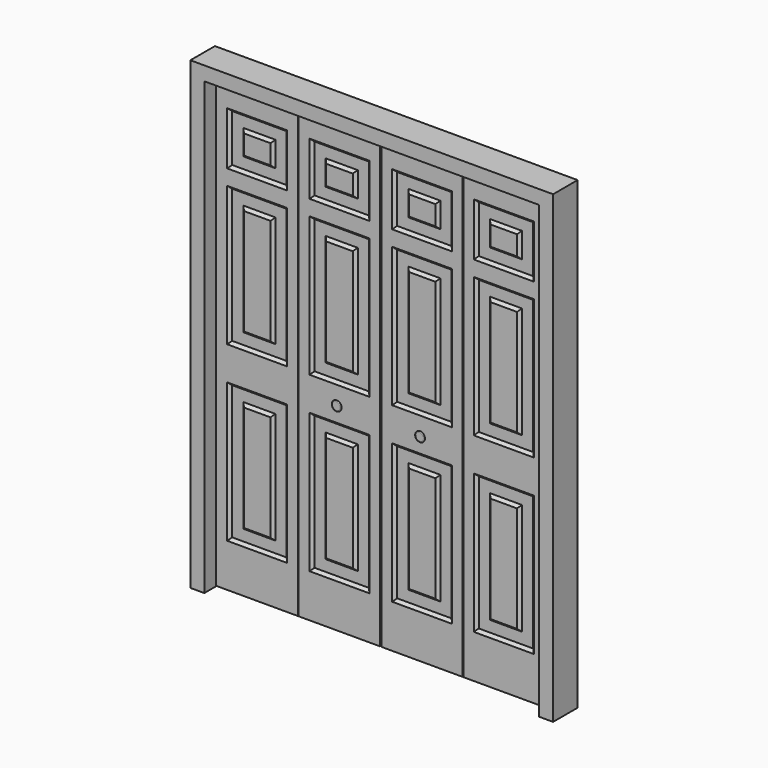
from build123d import *

# Parameters (mm, degrees)
F1_DEPTH  = 69.85
F0_W      = 1524
F0_H      = 2051.05
F2_DEPTH  = 19.05
F3_W      = 520.9721539497
F3_H      = 12.7
F4_DEPTH  = 88.901
F5_W      = 3.175
F5_H      = 2025.65
F7_DEPTH  = 88.901
F5_W_2    = 247.65
F5_H_2    = 215.9
F5_W_3    = 146.05
F5_H_3    = 114.3
F5_H_4    = 609.6
F5_H_5    = 508
F6_W      = 247.65
F6_H      = 215.9
F6_W_2    = 146.05
F6_H_2    = 114.3
F6_H_3    = 609.6
F6_H_4    = 508
F8_DEPTH  = 12.7
F9_SIZE   = 12.69999
F10_SIZE  = 12.69999
F11_R     = 6.35
F12_DEPTH = 12.7
F13_R     = 22.225
F14_DEPTH = 3.175
F15_R     = 6.35
F16_DEPTH = 12.7
F17_R     = 22.225
F18_DEPTH = 3.175


# Not quite as in the source:
# - a fillet or chamfer that OpenCascade refuses, or shapes differently, is made with other operations: its cross-section is extruded or revolved along the edge and cut away or added
# - a fillet or chamfer is up to 0.001 mm smaller than in the source, because OpenCascade refuses the exact size


with BuildPart() as f1:
    # F0 (on Front) → F1 (new body, symmetric)
    with BuildSketch(Plane.XZ):
        Polygon((825.5, 1057.275), (-825.5, 1057.275), (-825.5, -1057.275), (-762, -1057.275), (-762, 993.775), (762, 993.775), (762, -1057.275), (825.5, -1057.275), align=None)
    extrude(amount=F1_DEPTH, both=True)

    # F0 (on Front) → F2 (join, symmetric)
    with BuildSketch(Plane.XZ):
        with Locations((0, -31.75)):
            Rectangle(F0_W, F0_H)
    extrude(amount=F2_DEPTH, both=True)

    # F3 (on face) → F4 (cut, through all)
    with BuildSketch(Plane.XZ.offset(19.05)):
        Polygon((0, 981.075), (-3.175, 981.075), (-3.175, -1044.575), (0, -1044.575), (3.175, -1044.575), (3.175, 981.075), align=None)
        Polygon((-3.175, -1044.575), (-749.3, -1044.575), (-749.3, 981.075), (-683.8496296883, 981.075), (-683.8496296883, 993.775), (-762, 993.775), (-762, -1057.275), (762, -1057.275), (762, 993.775), (683.8496296883, 993.775), (683.8496296883, 981.075), (749.3, 981.075), (749.3, -1044.575), (3.175, -1044.575), (0, -1044.575), align=None)
        with Locations((410.6635527134, 987.425)):
            Rectangle(F3_W, F3_H)
        Polygon((-137.4774757385, 981.075), (-3.175, 981.075), (0, 981.075), (3.175, 981.075), (137.4774757385, 981.075), (137.4774757385, 993.775), (-137.4774757385, 993.775), align=None)
        with Locations((-410.6635527134, 987.425)):
            Rectangle(F3_W, F3_H)
    extrude(amount=-F4_DEPTH, mode=Mode.SUBTRACT)

    # F5 (on face) + F6 (on face) → F7 (cut, through all)
    with BuildSketch(Plane.XZ.offset(19.05)):
        with Locations((-374.65, -31.75)):
            Rectangle(F5_W, F5_H)
    with BuildSketch(Plane.XZ.offset(19.05)):
        Polygon((376.2375, 981.075), (373.0625, 981.075), (373.0625, -1044.575), (374.65, -1044.575), (376.2375, -1044.575), align=None)
    extrude(amount=-F7_DEPTH, mode=Mode.SUBTRACT)

    # F5 (on face) + F6 (on face) → F8 (cut)
    with BuildSketch(Plane.XZ.offset(19.05)):
        with Locations((-561.975, 765.175)):
            Rectangle(F5_W_2, F5_H_2)
        with Locations((-561.975, 765.175)):
            Rectangle(F5_W_3, F5_H_3, mode=Mode.SUBTRACT)
        with Locations((-561.975, 257.175)):
            Rectangle(F5_W_2, F5_H_4)
        with Locations((-561.975, 257.175)):
            Rectangle(F5_W_3, F5_H_5, mode=Mode.SUBTRACT)
        with Locations((-561.975, -530.225)):
            Rectangle(F5_W_2, F5_H_4)
        with Locations((-561.975, -530.225)):
            Rectangle(F5_W_3, F5_H_5, mode=Mode.SUBTRACT)
        with Locations((-187.325, -530.225)):
            Rectangle(F5_W_2, F5_H_4)
        with Locations((-187.325, -530.225)):
            Rectangle(F5_W_3, F5_H_5, mode=Mode.SUBTRACT)
        with Locations((-187.325, 257.175)):
            Rectangle(F5_W_2, F5_H_4)
        with Locations((-187.325, 257.175)):
            Rectangle(F5_W_3, F5_H_5, mode=Mode.SUBTRACT)
        with Locations((-187.325, 765.175)):
            Rectangle(F5_W_2, F5_H_2)
        with Locations((-187.325, 765.175)):
            Rectangle(F5_W_3, F5_H_3, mode=Mode.SUBTRACT)
    with BuildSketch(Plane.XZ.offset(19.05)):
        with Locations((188.9198460856, 765.175)):
            Rectangle(F6_W, F6_H)
        with Locations((188.9198460856, 765.175)):
            Rectangle(F6_W_2, F6_H_2, mode=Mode.SUBTRACT)
        with Locations((188.9198460856, 257.175)):
            Rectangle(F6_W, F6_H_3)
        with Locations((188.9198460856, 257.175)):
            Rectangle(F6_W_2, F6_H_4, mode=Mode.SUBTRACT)
        with Locations((188.9198460856, -530.225)):
            Rectangle(F6_W, F6_H_3)
        with Locations((188.9198460856, -530.225)):
            Rectangle(F6_W_2, F6_H_4, mode=Mode.SUBTRACT)
        with Locations((560.3801539144, -530.225)):
            Rectangle(F6_W, F6_H_3)
        with Locations((560.3801539144, -530.225)):
            Rectangle(F6_W_2, F6_H_4, mode=Mode.SUBTRACT)
        with Locations((560.3801539144, 257.175)):
            Rectangle(F6_W, F6_H_3)
        with Locations((560.3801539144, 257.175)):
            Rectangle(F6_W_2, F6_H_4, mode=Mode.SUBTRACT)
        with Locations((560.3801539144, 765.175)):
            Rectangle(F6_W, F6_H)
        with Locations((560.3801539144, 765.175)):
            Rectangle(F6_W_2, F6_H_2, mode=Mode.SUBTRACT)
    extrude(amount=-F8_DEPTH, mode=Mode.SUBTRACT)

    # F9 (size 12.7 in the source; OpenCascade refuses exactly that, so slightly less here)
    f9_edges = [f1.edges().sort_by_distance(p)[0] for p in [
        (-635, -19.05, 257.175),
        (-561.975, -19.05, 511.175),
        (-488.95, -19.05, 257.175),
        (-561.975, -19.05, 3.175),
        (-260.35, -19.05, 257.175),
        (-187.325, -19.05, 511.175),
        (-114.3, -19.05, 257.175),
        (-187.325, -19.05, 3.175),
        (-187.325, -19.05, 822.325),
        (-114.3, -19.05, 765.175),
        (-187.325, -19.05, 708.025),
        (-260.35, -19.05, 765.175),
        (-635, -19.05, 765.175),
        (-561.975, -19.05, 822.325),
        (-488.95, -19.05, 765.175),
        (-561.975, -19.05, 708.025),
        (-635, -19.05, -530.225),
        (-561.975, -19.05, -276.225),
        (-488.95, -19.05, -530.225),
        (-561.975, -19.05, -784.225),
        (-187.325, -19.05, -784.225),
        (-260.35, -19.05, -530.225),
        (-187.325, -19.05, -276.225),
        (-114.3, -19.05, -530.225),
        (188.919846, -19.05, -784.225),
        (115.894846, -19.05, -530.225),
        (188.919846, -19.05, -276.225),
        (261.944846, -19.05, -530.225),
        (261.944846, -19.05, 257.175),
        (188.919846, -19.05, 3.175),
        (115.894846, -19.05, 257.175),
        (188.919846, -19.05, 511.175),
        (560.380154, -19.05, -276.225),
        (633.405154, -19.05, -530.225),
        (560.380154, -19.05, -784.225),
        (487.355154, -19.05, -530.225),
        (560.380154, -19.05, 3.175),
        (487.355154, -19.05, 257.175),
        (560.380154, -19.05, 511.175),
        (633.405154, -19.05, 257.175),
        (560.380154, -19.05, 708.025),
        (487.355154, -19.05, 765.175),
        (560.380154, -19.05, 822.325),
        (633.405154, -19.05, 765.175),
        (188.919846, -19.05, 708.025),
        (115.894846, -19.05, 765.175),
        (188.919846, -19.05, 822.325),
        (261.944846, -19.05, 765.175),
    ]]
    chamfer(f9_edges, length=F9_SIZE)

    # F10 (size 12.7 in the source; OpenCascade refuses exactly that, so slightly less here)
    f10_edges = [f1.edges().sort_by_distance(p)[0] for p in [
        (560.380154, -19.05, 657.225),
        (436.555154, -19.05, 765.175),
        (560.380154, -19.05, 873.125),
        (684.205154, -19.05, 765.175),
        (560.380154, -19.05, 561.975),
        (436.555154, -19.05, 257.175),
        (684.205154, -19.05, 257.175),
        (560.380154, -19.05, -47.625),
        (560.380154, -19.05, -225.425),
        (436.555154, -19.05, -530.225),
        (684.205154, -19.05, -530.225),
        (560.380154, -19.05, -835.025),
        (188.919846, -19.05, -835.025),
        (312.744846, -19.05, -530.225),
        (65.094846, -19.05, -530.225),
        (188.919846, -19.05, -225.425),
        (-187.325, -19.05, -225.425),
        (-63.5, -19.05, -530.225),
        (-311.15, -19.05, -530.225),
        (-187.325, -19.05, -835.025),
        (-561.975, -19.05, -835.025),
        (-685.8, -19.05, -530.225),
        (-438.15, -19.05, -530.225),
        (-561.975, -19.05, -225.425),
        (-561.975, -19.05, -47.625),
        (-685.8, -19.05, 257.175),
        (-438.15, -19.05, 257.175),
        (-561.975, -19.05, 561.975),
        (-187.325, -19.05, 561.975),
        (-311.15, -19.05, 257.175),
        (-63.5, -19.05, 257.175),
        (-685.8, -19.05, 765.175),
        (-561.975, -19.05, 657.225),
        (-438.15, -19.05, 765.175),
        (-311.15, -19.05, 765.175),
        (-187.325, -19.05, 657.225),
        (-63.5, -19.05, 765.175),
        (-187.325, -19.05, -47.625),
        (65.094846, -19.05, 257.175),
        (188.919846, -19.05, -47.625),
        (312.744846, -19.05, 257.175),
        (188.919846, -19.05, 561.975),
        (188.919846, -19.05, 657.225),
        (65.094846, -19.05, 765.175),
        (188.919846, -19.05, 873.125),
        (312.744846, -19.05, 765.175),
        (-187.325, -19.05, 873.125),
        (-561.975, -19.05, 873.125),
    ]]
    chamfer(f10_edges, length=F10_SIZE)

    # F11 (on face) → F12 (join)
    with BuildSketch(Plane.XZ.offset(19.05)):
        with Locations((-189.70625, -136.525)):
            Circle(F11_R)
    extrude(amount=F12_DEPTH)

    # F13 (on face) → F14 (join)
    with BuildSketch(Plane.XZ.offset(31.75)):
        with Locations((-189.70625, -136.525)):
            Circle(F13_R)
    extrude(amount=F14_DEPTH)

    # F15 (on face) → F16 (join)
    with BuildSketch(Plane.XZ.offset(19.05)):
        with Locations((189.7126, -136.525)):
            Circle(F15_R)
    extrude(amount=F16_DEPTH)

    # F17 (on face) → F18 (join)
    with BuildSketch(Plane.XZ.offset(31.75)):
        with Locations((189.7126, -136.525)):
            Circle(F17_R)
    extrude(amount=F18_DEPTH)

    # F19: fillet of radius 5.08 on 2 edges, made by hand

    # F19_s1 → F19_t2 (revolve, cut)
    with BuildSketch(Plane.XY.offset(-136.525)):
        with BuildLine():
            ThreePointArc((-167.48125, -31.75), (-169.3507297079, -34.0571134838), (-172.1905360393, -34.925))
            Line((-172.1905360393, -34.925), (-167.48125, -34.925))
            Line((-167.48125, -34.925), (-167.48125, -31.75))
        make_face()
    revolve(axis=Axis((-189.70625, -34.925, -136.525), (0, -1, 0)), mode=Mode.SUBTRACT)

    # F19_s3 → F19_t4 (revolve, cut)
    with BuildSketch(Plane.XY.offset(-136.525)):
        with BuildLine():
            ThreePointArc((211.9376, -31.75), (210.0681202921, -34.0571134838), (207.2283139607, -34.925))
            Line((207.2283139607, -34.925), (211.9376, -34.925))
            Line((211.9376, -34.925), (211.9376, -31.75))
        make_face()
    revolve(axis=Axis((189.7126, -34.925, -136.525), (0, -1, 0)), mode=Mode.SUBTRACT)


solid = f1.part
